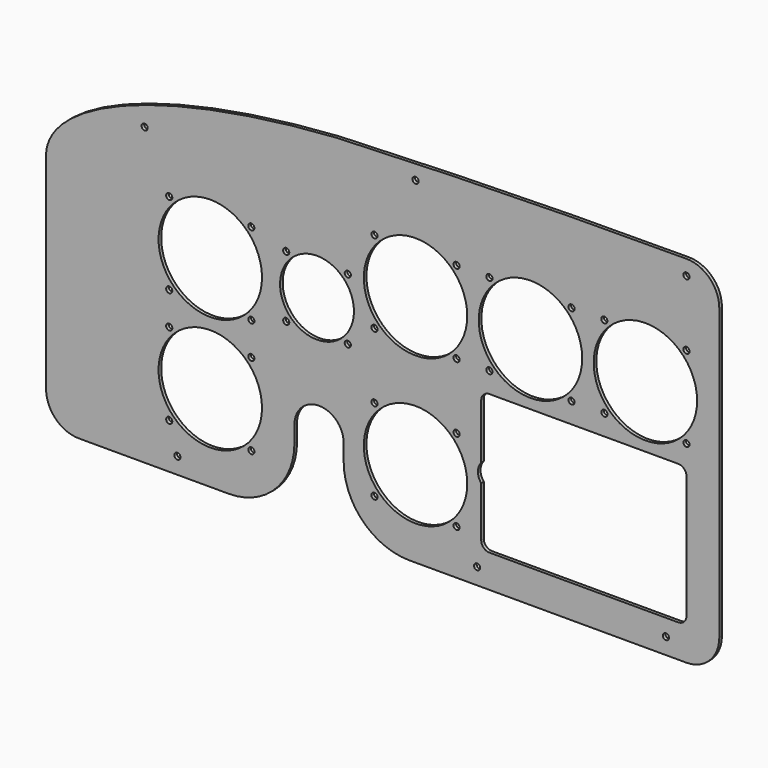
from build123d import *

# Parameters (mm, degrees)
F0_R     = 2.38125
F1_DEPTH = 2.54
F2_R     = 40.005
F2_R_2   = 28.575
F2_R_3   = 2.38125
F3_DEPTH = 2.5410001


with BuildPart() as f1:
    # F0 (on Front) → F1 (new body)
    with BuildSketch(Plane.XZ):
        with BuildLine():
            ThreePointArc((6.3499999233, -24.9008008357), (-1.0762466814, -6.9535395158), (-19.0125346344, 0.4991715332))
            ThreePointArc((-19.0125346344, 0.4991715332), (-154.4493523287, -0.8097271588), (-289.8234049708, -5.1353108434))
            add(Edge.make_bspline(
                [(-289.8234049708, -5.1353108434), (-514.6487503932, -20.2006873557), (-514.3499970436, -90.5002)],
                knots=[4.9283667006, 4.9283667006, 4.9283667006, 6.2844832596, 6.2844832596, 6.2844832596], degree=2, weights=[1, 0.7787921925, 1]))
            Line((-514.3499970436, -90.5002), (-514.3499970436, -249.2502))
            ThreePointArc((-514.3499970436, -249.2502), (-506.9105092857, -267.2107122421), (-488.9499970436, -274.6502))
            Line((-488.9499970436, -274.6502), (-373.0752, -274.6502))
            ThreePointArc((-373.0752, -274.6502), (-337.1541755157, -259.7712244843), (-322.2752, -223.8502))
            Line((-322.2752, -223.8502), (-322.2752, -211.0369156084))
            ThreePointArc((-322.2752, -211.0369156084), (-303.2252, -191.9869156084), (-284.1752, -211.0369156084))
            Line((-284.1752, -211.0369156084), (-284.1752, -223.7369156084))
            ThreePointArc((-284.1752, -223.7369156084), (-269.2962244843, -259.6579400927), (-233.3752, -274.5369156084))
            Line((-233.3752, -274.5369156084), (-19.0500000767, -274.5369156084))
            ThreePointArc((-19.0500000767, -274.5369156084), (-1.0894878346, -267.0974278505), (6.3499999233, -249.1369156084))
            Line((6.3499999233, -249.1369156084), (6.3499999233, -24.9008008357))
        make_face()
        with Locations((-412.75, -261.9502)):
            Circle(F0_R, mode=Mode.SUBTRACT)
        with Locations((-180.975, -261.9502)):
            Circle(F0_R, mode=Mode.SUBTRACT)
        with Locations((-34.925, -261.9502)):
            Circle(F0_R, mode=Mode.SUBTRACT)
        with BuildLine():
            ThreePointArc((-177.8000000767, -147.5369156084), (-175.9401281373, -143.0467875478), (-171.4500000767, -141.1869156084))
            Line((-171.4500000767, -141.1869156084), (-25.4000000767, -141.1869156084))
            ThreePointArc((-25.4000000767, -141.1869156084), (-20.9098720162, -143.0467875478), (-19.0500000767, -147.5369156084))
            Line((-19.0500000767, -147.5369156084), (-19.0500000767, -242.7869156084))
            ThreePointArc((-19.0500000767, -242.7869156084), (-20.9098720162, -247.2770436689), (-25.4000000767, -249.1369156084))
            Line((-25.4000000767, -249.1369156084), (-171.4500000767, -249.1369156084))
            ThreePointArc((-171.4500000767, -249.1369156084), (-175.9401281373, -247.2770436689), (-177.8000000767, -242.7869156084))
            Line((-177.8000000767, -242.7869156084), (-177.8000000767, -203.9237609675))
            ThreePointArc((-177.8000000767, -203.9237609675), (-180.3400000767, -196.9399156084), (-177.8000000767, -189.9560702493))
            Line((-177.8000000767, -189.9560702493), (-177.8000000767, -147.5369156084))
        make_face(mode=Mode.SUBTRACT)
        with Locations((-438.15, -46.0502)):
            Circle(F0_R, mode=Mode.SUBTRACT)
        with Locations((-228.6, -14.1869156084)):
            Circle(F0_R, mode=Mode.SUBTRACT)
        with Locations((-19.05, -11.1252)):
            Circle(F0_R, mode=Mode.SUBTRACT)
    extrude(amount=F1_DEPTH)

    # F2 (on face) → F3 (cut, through all)
    with BuildSketch(Plane.XZ.offset(2.54)):
        with Locations((-50.8, -93.5619156084)):
            Circle(F2_R)
        with Locations((-139.7, -93.5619156084)):
            Circle(F2_R)
        with Locations((-228.6, -93.5619156084)):
            Circle(F2_R)
        with Locations((-304.8, -118.9619156084)):
            Circle(F2_R_2)
        with Locations((-19.05, -125.3119156084)):
            Circle(F2_R_3)
        with Locations((-82.5499999959, -125.3119156124)):
            Circle(F2_R_3)
        with Locations((-82.5500000081, -61.8119156165)):
            Circle(F2_R_3)
        with Locations((-19.0500000122, -61.8119155962)):
            Circle(F2_R_3)
        with Locations((-280.9748, -142.7871156084)):
            Circle(F2_R_3)
        with Locations((-280.9748, -95.1367156084)):
            Circle(F2_R_3)
        with Locations((-328.6252, -95.1367156084)):
            Circle(F2_R_3)
        with Locations((-328.6252, -142.7871156084)):
            Circle(F2_R_3)
        with Locations((-228.6, -207.8619156084)):
            Circle(F2_R)
        with Locations((-387.35, -118.9619156084)):
            Circle(F2_R)
        with Locations((-387.35, -207.8619156084)):
            Circle(F2_R)
        with Locations((-171.4499999959, -125.3119156124)):
            Circle(F2_R_3)
        with Locations((-107.95, -125.3119156084)):
            Circle(F2_R_3)
        with Locations((-107.9500000122, -61.8119155962)):
            Circle(F2_R_3)
        with Locations((-171.4500000081, -61.8119156165)):
            Circle(F2_R_3)
        with Locations((-260.3499999959, -125.3119156124)):
            Circle(F2_R_3)
        with Locations((-196.85, -125.3119156084)):
            Circle(F2_R_3)
        with Locations((-196.8500000122, -61.8119155962)):
            Circle(F2_R_3)
        with Locations((-260.3500000081, -61.8119156165)):
            Circle(F2_R_3)
        with Locations((-260.3500000081, -176.1119156165)):
            Circle(F2_R_3)
        with Locations((-260.3499999959, -239.6119156124)):
            Circle(F2_R_3)
        with Locations((-196.8500000122, -176.1119155962)):
            Circle(F2_R_3)
        with Locations((-196.85, -239.6119156084)):
            Circle(F2_R_3)
        with Locations((-419.1000000081, -176.1119156165)):
            Circle(F2_R_3)
        with Locations((-355.6000000122, -176.1119155962)):
            Circle(F2_R_3)
        with Locations((-355.6, -239.6119156084)):
            Circle(F2_R_3)
        with Locations((-419.0999999959, -239.6119156124)):
            Circle(F2_R_3)
        with Locations((-355.6, -150.7119156084)):
            Circle(F2_R_3)
        with Locations((-419.1000000081, -87.2119156165)):
            Circle(F2_R_3)
        with Locations((-355.6000000122, -87.2119155962)):
            Circle(F2_R_3)
        with Locations((-419.0999999959, -150.7119156124)):
            Circle(F2_R_3)
    extrude(amount=-F3_DEPTH, mode=Mode.SUBTRACT)


solid = f1.part
